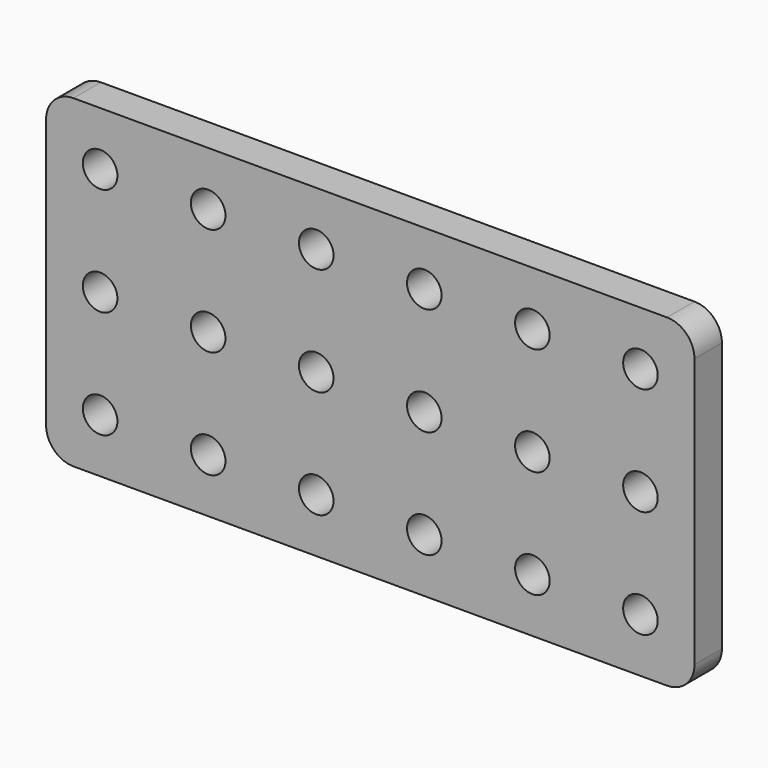
from build123d import *

# Parameters (mm, degrees)
F0_R     = 1.6
F1_DEPTH = 3.175


# Not quite as in the source:
# - a length typed as a fraction of an inch, garbled in the dataset ("3 / 203.2 mm" for 3/8 in), is restored


with BuildPart() as f1:
    # F0 (on Front) → F1 (new body)
    with BuildSketch(Plane.XZ):
        with BuildLine():
            Line((57.46, 0), (2.54, 0))
            ThreePointArc((2.54, 0), (0.7439487758, -0.7439487758), (0, -2.54))
            Line((0, -2.54), (0, -27.46))
            ThreePointArc((0, -27.46), (0.7439487758, -29.2560512242), (2.54, -30))
            Line((2.54, -30), (57.46, -30))
            ThreePointArc((57.46, -30), (59.2560512242, -29.2560512242), (60, -27.46))
            Line((60, -27.46), (60, -2.54))
            ThreePointArc((60, -2.54), (59.2560512242, -0.7439487758), (57.46, 0))
        make_face()
        with Locations((5, -25)):
            Circle(F0_R, mode=Mode.SUBTRACT)
        with Locations((15, -25)):
            Circle(F0_R, mode=Mode.SUBTRACT)
        with Locations((25, -25)):
            Circle(F0_R, mode=Mode.SUBTRACT)
        with Locations((35, -25)):
            Circle(F0_R, mode=Mode.SUBTRACT)
        with Locations((45, -25)):
            Circle(F0_R, mode=Mode.SUBTRACT)
        with Locations((55, -25)):
            Circle(F0_R, mode=Mode.SUBTRACT)
        with Locations((5, -15)):
            Circle(F0_R, mode=Mode.SUBTRACT)
        with Locations((15, -15)):
            Circle(F0_R, mode=Mode.SUBTRACT)
        with Locations((25, -15)):
            Circle(F0_R, mode=Mode.SUBTRACT)
        with Locations((5, -5)):
            Circle(F0_R, mode=Mode.SUBTRACT)
        with Locations((15, -5)):
            Circle(F0_R, mode=Mode.SUBTRACT)
        with Locations((25, -5)):
            Circle(F0_R, mode=Mode.SUBTRACT)
        with Locations((35, -15)):
            Circle(F0_R, mode=Mode.SUBTRACT)
        with Locations((45, -15)):
            Circle(F0_R, mode=Mode.SUBTRACT)
        with Locations((55, -15)):
            Circle(F0_R, mode=Mode.SUBTRACT)
        with Locations((35, -5)):
            Circle(F0_R, mode=Mode.SUBTRACT)
        with Locations((45, -5)):
            Circle(F0_R, mode=Mode.SUBTRACT)
        with Locations((55, -5)):
            Circle(F0_R, mode=Mode.SUBTRACT)
    extrude(amount=F1_DEPTH)


solid = f1.part
